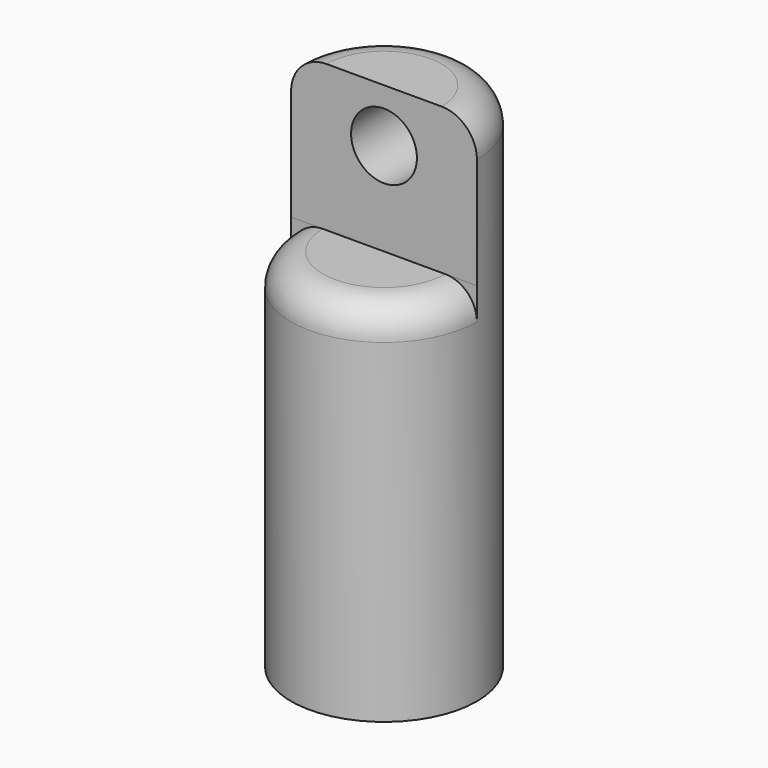
from build123d import *

# Parameters (mm, degrees)
F0_R        = 6.35
F1_DEPTH    = 25
F3_DEPTH    = 12.7
F4_R        = 2.25
F5_DEPTH    = 25
F6_W        = 18.3003712445
F6_H        = 9.7342398949
F7_DEPTH    = 2.7
F8_T2_ANGLE = 289.0918893802
F9_T2_ANGLE = 180


# Not quite as in the source:
# - a fillet or chamfer that OpenCascade refuses, or shapes differently, is made with other operations: its cross-section is extruded or revolved along the edge and cut away or added


with BuildPart() as f1:
    # F0 (on Top) → F1 (new body)
    with BuildSketch(Plane.XY):
        Circle(F0_R)
    extrude(amount=F1_DEPTH)

    # F2 (on face) → F3 (join)
    with BuildSketch(Plane.XY.offset(25)):
        with BuildLine():
            Line((-6.35, 0), (6.35, 0))
            ThreePointArc((6.35, 0), (0, 6.35), (-6.35, 0))
        make_face()
    extrude(amount=F3_DEPTH)

    # F4 (on face) → F5 (cut)
    with BuildSketch(Plane.XZ):
        with Locations((0, 31.35)):
            Circle(F4_R)
    extrude(amount=-F5_DEPTH, mode=Mode.SUBTRACT)

    # F6 (on face) → F7 (cut)
    with BuildSketch(Plane.XY.offset(37.7)):
        with Locations((0, 3.4640058875)):
            Rectangle(F6_W, F6_H)
    extrude(amount=-F7_DEPTH, mode=Mode.SUBTRACT)

    # F8: fillet of radius 2.4142135624 on 1 edges, made by hand

    # F8_s1 → F8_t2 (revolve, cut)
    with BuildSketch(Plane(origin=(0, 0, 0), x_dir=(0, 0, 1), z_dir=(0.8145809142, -0.5800499411, 0))):
        with BuildLine():
            ThreePointArc((32.5857864376, 6.35), (34.2928932188, 5.6428932188), (35, 3.9357864376))
            Line((35, 3.9357864376), (35, 6.35))
            Line((35, 6.35), (32.5857864376, 6.35))
        make_face()
    revolve(axis=Axis((0, 0, 35), (0, 0, -1)), revolution_arc=F8_T2_ANGLE, mode=Mode.SUBTRACT)

    # F9: fillet of radius 2.1727922061 on 1 edges, made by hand

    # F9_s1 → F9_t2 (revolve, cut)
    with BuildSketch(Plane.XZ):
        with BuildLine():
            ThreePointArc((-6.35, 22.8272077939), (-5.7136038969, 24.3636038969), (-4.1772077939, 25))
            Line((-4.1772077939, 25), (-6.35, 25))
            Line((-6.35, 25), (-6.35, 22.8272077939))
        make_face()
    revolve(axis=Axis((0, 0, 25), (0, 0, 1)), revolution_arc=F9_T2_ANGLE, mode=Mode.SUBTRACT)


solid = f1.part
